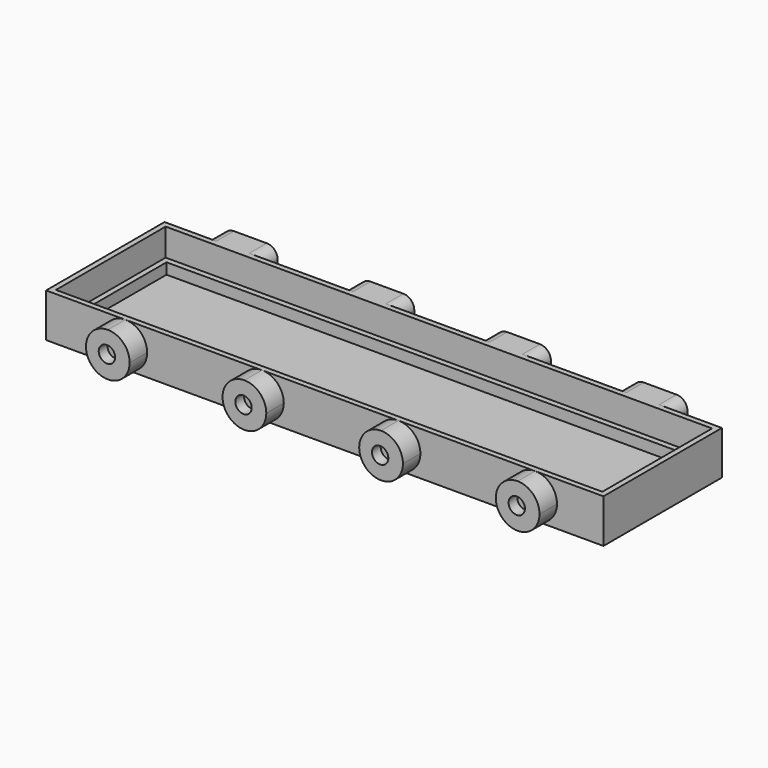
from build123d import *

# Parameters (mm, degrees)
F0_W      = 102
F0_H      = 27.1
F0_W_2    = 100
F0_H_2    = 25.1
F1_DEPTH  = 8
F2_DEPTH  = 1
F3_W      = 100
F3_H      = 25.1
F3_W_2    = 98
F3_H_2    = 23
F4_DEPTH  = 2
F6_DEPTH  = 4
F7_R      = 1.5
F8_DEPTH  = 2
F10_DEPTH = 4
F11_R     = 1.5
F12_DEPTH = 2


# Not quite as in the source:
# - a feature names something its author has since deleted; it is built from what else it names


with BuildPart() as f1:
    # F0 (on Top) → F1 (new body)
    with BuildSketch(Plane.XY):
        Rectangle(F0_W, F0_H)
        Rectangle(F0_W_2, F0_H_2, mode=Mode.SUBTRACT)
    extrude(amount=F1_DEPTH)

    # F0 (on Top) → F2 (join)
    with BuildSketch(Plane.XY):
        Rectangle(F0_W_2, F0_H_2)
    extrude(amount=F2_DEPTH)

    # F3 (on face) → F4 (join)
    with BuildSketch(Plane.XY.offset(1)):
        Rectangle(F3_W, F3_H)
        Rectangle(F3_W_2, F3_H_2, mode=Mode.SUBTRACT)
    extrude(amount=F4_DEPTH)

    # F5 (on face) → F6 (join)
    with BuildSketch(Plane.XZ.offset(13.55)):
        with BuildLine():
            ThreePointArc((-36.5, 0), (-33.6715728753, 1.1715728753), (-32.5, 4))
            ThreePointArc((-32.5, 4), (-33.6715728968, 6.8284271463), (-36.5000000611, 8))
            ThreePointArc((-36.5000000611, 8), (-40.5, 3.9999999695), (-36.5, 0))
        make_face()
        with BuildLine():
            ThreePointArc((-7.5, 4), (-8.6715728753, 6.8284271247), (-11.5, 8))
            ThreePointArc((-11.5, 8), (-15.5, 4), (-11.5, 0))
            ThreePointArc((-11.5, 0), (-8.6715728753, 1.1715728753), (-7.5, 4))
        make_face()
        with BuildLine():
            ThreePointArc((17.5, 4), (16.3284271247, 6.8284271247), (13.5, 8))
            ThreePointArc((13.5, 8), (9.5, 4.0000000201), (13.4999999598, 0))
            ThreePointArc((13.4999999598, 0), (16.3284271105, 1.171572861), (17.5, 4))
        make_face()
        with BuildLine():
            ThreePointArc((42.5, 4), (41.3284271247, 6.8284271247), (38.5, 8))
            ThreePointArc((38.5, 8), (34.5, 4.0000000325), (38.499999935, 0))
            ThreePointArc((38.499999935, 0), (41.3284271017, 1.1715728523), (42.5, 4))
        make_face()
    extrude(amount=F6_DEPTH)

    # F7 (on face) → F8 (cut)
    with BuildSketch(Plane.XZ.offset(17.55)):
        with Locations((-36.6656929255, 4)):
            Circle(F7_R)
        with Locations((-11.6656929255, 4)):
            Circle(F7_R)
        with Locations((13.3343070745, 4)):
            Circle(F7_R)
        with Locations((38.3343070745, 4)):
            Circle(F7_R)
    extrude(amount=-F8_DEPTH, mode=Mode.SUBTRACT)

    # F9 (on face) → F10 (join)
    with BuildSketch(Plane(origin=(0, 13.55, 0), x_dir=(-1, 0, 0), z_dir=(0, 1, 0))):
        with BuildLine():
            Line((-39.5, 0), (-33.5, 0))
            ThreePointArc((-33.5, 0), (-32.0857864376, 0.5857864376), (-31.5, 2))
            Line((-31.5, 2), (-31.5, 6))
            ThreePointArc((-31.5, 6), (-32.0857864376, 7.4142135624), (-33.5, 8))
            Line((-33.5, 8), (-39.5, 8))
            ThreePointArc((-39.5, 8), (-40.9142135624, 7.4142135624), (-41.5, 6))
            Line((-41.5, 6), (-41.5, 2))
            ThreePointArc((-41.5, 2), (-40.9142135624, 0.5857864376), (-39.5, 0))
        make_face()
        with BuildLine():
            ThreePointArc((-16.5, 2), (-15.9142135624, 0.5857864376), (-14.5, 0))
            Line((-14.5, 0), (-8.5, 0))
            ThreePointArc((-8.5, 0), (-7.0857864376, 0.5857864376), (-6.5, 2))
            Line((-6.5, 2), (-6.5, 6))
            ThreePointArc((-6.5, 6), (-7.0857864376, 7.4142135624), (-8.5, 8))
            Line((-8.5, 8), (-14.5, 8))
            ThreePointArc((-14.5, 8), (-15.9142135624, 7.4142135624), (-16.5, 6))
            Line((-16.5, 6), (-16.5, 2))
        make_face()
        with BuildLine():
            ThreePointArc((8.5, 2), (9.0857864376, 0.5857864376), (10.5, 0))
            Line((10.5, 0), (16.5, 0))
            ThreePointArc((16.5, 0), (17.9142135624, 0.5857864376), (18.5, 2))
            Line((18.5, 2), (18.5, 6))
            ThreePointArc((18.5, 6), (17.9142135624, 7.4142135624), (16.5, 8))
            Line((16.5, 8), (10.5, 8))
            ThreePointArc((10.5, 8), (9.0857864376, 7.4142135624), (8.5, 6))
            Line((8.5, 6), (8.5, 2))
        make_face()
        with BuildLine():
            ThreePointArc((33.5, 2), (34.0857864376, 0.5857864376), (35.5, 0))
            Line((35.5, 0), (41.5, 0))
            ThreePointArc((41.5, 0), (42.9142135624, 0.5857864376), (43.5, 2))
            Line((43.5, 2), (43.5, 6))
            ThreePointArc((43.5, 6), (42.9142135624, 7.4142135624), (41.5, 8))
            Line((41.5, 8), (35.5, 8))
            ThreePointArc((35.5, 8), (34.0857864376, 7.4142135624), (33.5, 6))
            Line((33.5, 6), (33.5, 2))
        make_face()
    extrude(amount=F10_DEPTH)

    # F11 (on face) → F12 (cut)
    with BuildSketch(Plane(origin=(0, 17.55, 0), x_dir=(-1, 0, 0), z_dir=(0, 1, 0))):
        with Locations((-36.5, 4)):
            Circle(F11_R)
        with Locations((-11.5, 4)):
            Circle(F11_R)
        with Locations((13.5, 4)):
            Circle(F11_R)
        with Locations((38.5, 4)):
            Circle(F11_R)
    extrude(amount=-F12_DEPTH, mode=Mode.SUBTRACT)


solid = f1.part
